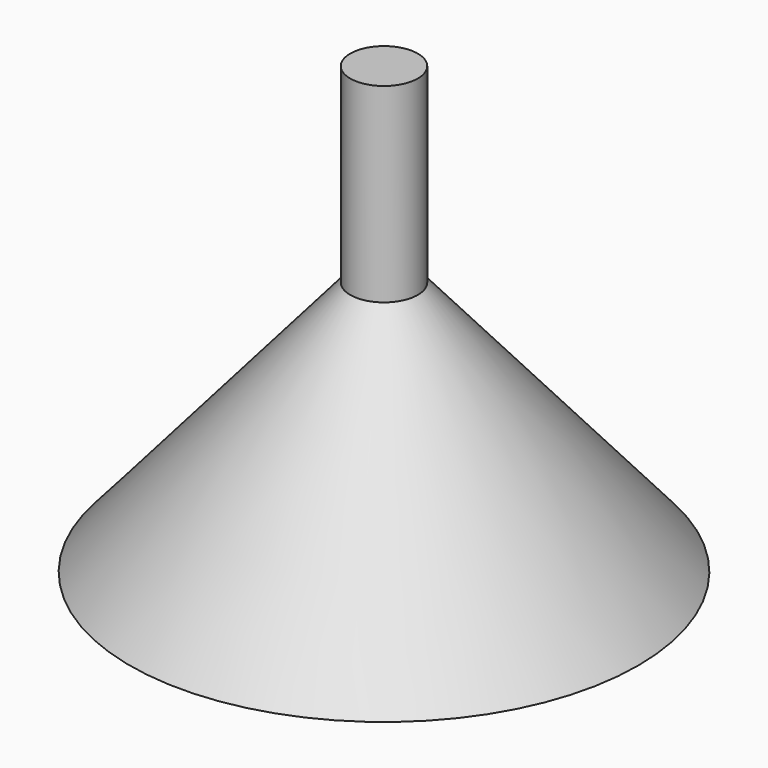
from build123d import *

# Parameters (mm, degrees)
F2_T     = 1.2
F4_D     = 300
F4_DEPTH = 1.201


with BuildPart() as f1:
    # F0 (on Front) → F1 (revolve)
    with BuildSketch(Plane.XZ):
        Polygon((-3.6914059892, 36.4218764007), (-35.1914092898, 0), (0, 0), (0, 63.2460936904), (-3.6914059892, 63.2460936904), align=None)
    revolve(axis=Axis((0, 0, 31.6230468452), (0, 0, -1)))

    # F2 (hollow, outwards: the wall grows on the outside; the body as it was is the cavity)
    f2_inside = f1.part
    offset(amount=F2_T, kind=Kind.INTERSECTION)
    add(f2_inside, mode=Mode.SUBTRACT)

    # F4 (through all, one way)
    with BuildSketch(Plane.XY):
        with Locations((0, 0)):
            Circle(F4_D / 2)
    extrude(amount=-F4_DEPTH, mode=Mode.SUBTRACT)


solid = f1.part
